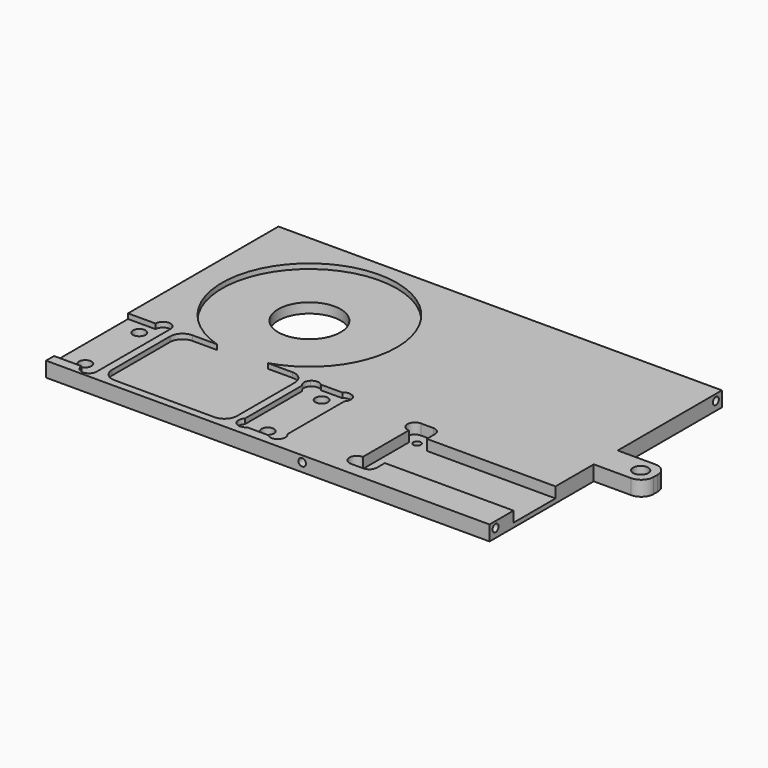
from build123d import *

# Parameters (mm, degrees)
F0_W      = 20
F0_H      = 12
F0_R      = 3
F1_DEPTH  = 6
F0_R_2    = 12.5
F0_R_3    = 2.5
F2_DEPTH  = 4
F3_DEPTH  = 2
F4_DEPTH  = 3
F0_R_4    = 1.5
F5_DEPTH  = 1.75
F6_R      = 1.5
F7_DEPTH  = 8
F8_R      = 1.5
F9_DEPTH  = 8
F10_R     = 1.5
F11_DEPTH = 5
F12_R     = 1.5
F13_DEPTH = 5
F14_R     = 5


# Not quite as in the source:
# - a feature names something its author has since deleted; it is built from what else it names


with BuildPart() as f1:
    # F0 (on Top) → F1 (new body)
    with BuildSketch(Plane.XY):
        with BuildLine():
            Line((0, 4), (0, 0))
            Line((0, 0), (177.5, 0))
            Line((177.5, 0), (177.5, 5))
            Line((177.5, 5), (177.5, 12))
            Line((177.5, 12), (126, 12))
            Line((126, 12), (126, 8))
            ThreePointArc((126, 8), (125.1213203436, 5.8786796564), (123, 5))
            Line((123, 5), (118, 5))
            ThreePointArc((118, 5), (115, 8), (118, 11))
            Line((118, 11), (118, 34))
            ThreePointArc((118, 34), (115, 37), (118, 40))
            Line((118, 40), (123, 40))
            ThreePointArc((123, 40), (125.1213203436, 39.1213203436), (126, 37))
            Line((126, 37), (126, 33))
            Line((126, 33), (177.5, 33))
            Line((177.5, 33), (177.5, 40))
            Line((177.5, 40), (177.5, 52.125))
            Line((177.5, 52.125), (177.5, 64.125))
            Line((177.5, 64.125), (177.5, 116.25))
            Line((177.5, 116.25), (0, 116.25))
            Line((0, 116.25), (0, 41))
            Line((0, 41), (11, 41))
            ThreePointArc((11, 41), (14, 44), (17, 41))
            Line((17, 41), (17, 4))
            ThreePointArc((17, 4), (14, 1), (11, 4))
            Line((11, 4), (0, 4))
        make_face()
        with BuildLine():
            Line((73, 8.2426406871), (73, 36.7573593129))
            ThreePointArc((73, 36.7573593129), (72.1213203436, 38.8786796564), (73, 41))
            ThreePointArc((73, 41), (75.1213203436, 41.8786796564), (77.2426406871, 41))
            Line((77.2426406871, 41), (85.7573593129, 41))
            ThreePointArc((85.7573593129, 41), (87.8786796564, 41.8786796564), (90, 41))
            ThreePointArc((90, 41), (90.8786796564, 38.8786796564), (90, 36.7573593129))
            Line((90, 36.7573593129), (90, 8.2426406871))
            ThreePointArc((90, 8.2426406871), (90.8786796564, 6.1213203436), (90, 4))
            ThreePointArc((90, 4), (87.8786796564, 3.1213203436), (85.7573593129, 4))
            Line((85.7573593129, 4), (77.2426406871, 4))
            ThreePointArc((77.2426406871, 4), (75.1213203436, 3.1213203436), (73, 4))
            ThreePointArc((73, 4), (72.1213203436, 6.1213203436), (73, 8.2426406871))
        make_face(mode=Mode.SUBTRACT)
        with BuildLine():
            ThreePointArc((34.8634325336, 42), (24.1407078419, 103.6049805312), (80, 75.5))
            ThreePointArc((80, 75.5), (73.1049805312, 54.6407078419), (55.1365674664, 42))
            Line((55.1365674664, 42), (65, 42))
            ThreePointArc((65, 42), (68.5355339059, 40.5355339059), (70, 37))
            Line((70, 37), (70, 8))
            ThreePointArc((70, 8), (68.5355339059, 4.4644660941), (65, 3))
            Line((65, 3), (25, 3))
            ThreePointArc((25, 3), (21.4644660941, 4.4644660941), (20, 8))
            Line((20, 8), (20, 37))
            ThreePointArc((20, 37), (21.4644660941, 40.5355339059), (25, 42))
            Line((25, 42), (34.8634325336, 42))
        make_face(mode=Mode.SUBTRACT)
        with Locations((187.5, 58.125)):
            Rectangle(F0_W, F0_H)
        with Locations((191.5, 58.125)):
            Circle(F0_R, mode=Mode.SUBTRACT)
    extrude(amount=F1_DEPTH)

    # F0 (on Top) → F2 (join)
    with BuildSketch(Plane.XY):
        with BuildLine():
            Line((55.1365674664, 42), (34.8634325336, 42))
            ThreePointArc((34.8634325336, 42), (45, 40.5), (55.1365674664, 42))
        make_face()
        with BuildLine():
            ThreePointArc((55.1365674664, 42), (73.1049805312, 54.6407078419), (80, 75.5))
            ThreePointArc((80, 75.5), (24.1407078419, 103.6049805312), (34.8634325336, 42))
            Line((34.8634325336, 42), (55.1365674664, 42))
        make_face()
        with Locations((45, 75.5)):
            Circle(F0_R_2, mode=Mode.SUBTRACT)
        with BuildLine():
            Line((0, 41), (0, 4))
            Line((0, 4), (11, 4))
            ThreePointArc((11, 4), (14, 1), (17, 4))
            Line((17, 4), (17, 41))
            ThreePointArc((17, 41), (14, 44), (11, 41))
            Line((11, 41), (0, 41))
        make_face()
        with Locations((8.5, 9)):
            Circle(F0_R_3, mode=Mode.SUBTRACT)
        with Locations((8.5, 36)):
            Circle(F0_R_3, mode=Mode.SUBTRACT)
        with BuildLine():
            ThreePointArc((73, 41), (72.1213203436, 38.8786796564), (73, 36.7573593129))
            Line((73, 36.7573593129), (73, 8.2426406871))
            ThreePointArc((73, 8.2426406871), (72.1213203436, 6.1213203436), (73, 4))
            ThreePointArc((73, 4), (75.1213203436, 3.1213203436), (77.2426406871, 4))
            Line((77.2426406871, 4), (85.7573593129, 4))
            ThreePointArc((85.7573593129, 4), (87.8786796564, 3.1213203436), (90, 4))
            ThreePointArc((90, 4), (90.8786796564, 6.1213203436), (90, 8.2426406871))
            Line((90, 8.2426406871), (90, 36.7573593129))
            ThreePointArc((90, 36.7573593129), (90.8786796564, 38.8786796564), (90, 41))
            ThreePointArc((90, 41), (87.8786796564, 41.8786796564), (85.7573593129, 41))
            Line((85.7573593129, 41), (77.2426406871, 41))
            ThreePointArc((77.2426406871, 41), (75.1213203436, 41.8786796564), (73, 41))
        make_face()
        with Locations((81.5, 9)):
            Circle(F0_R_3, mode=Mode.SUBTRACT)
        with Locations((81.5, 36)):
            Circle(F0_R_3, mode=Mode.SUBTRACT)
        with BuildLine():
            ThreePointArc((55.1365674664, 42), (45, 40.5), (34.8634325336, 42))
            Line((34.8634325336, 42), (25, 42))
            ThreePointArc((25, 42), (21.4644660941, 40.5355339059), (20, 37))
            Line((20, 37), (20, 8))
            ThreePointArc((20, 8), (21.4644660941, 4.4644660941), (25, 3))
            Line((25, 3), (65, 3))
            ThreePointArc((65, 3), (68.5355339059, 4.4644660941), (70, 8))
            Line((70, 8), (70, 37))
            ThreePointArc((70, 37), (68.5355339059, 40.5355339059), (65, 42))
            Line((65, 42), (55.1365674664, 42))
        make_face()
    extrude(amount=F2_DEPTH)

    # F0 (on Top) → F3 (join)
    with BuildSketch(Plane.XY):
        with BuildLine():
            ThreePointArc((55.1365674664, 42), (45, 40.5), (34.8634325336, 42))
            Line((34.8634325336, 42), (25, 42))
            ThreePointArc((25, 42), (21.4644660941, 40.5355339059), (20, 37))
            Line((20, 37), (20, 8))
            ThreePointArc((20, 8), (21.4644660941, 4.4644660941), (25, 3))
            Line((25, 3), (65, 3))
            ThreePointArc((65, 3), (68.5355339059, 4.4644660941), (70, 8))
            Line((70, 8), (70, 37))
            ThreePointArc((70, 37), (68.5355339059, 40.5355339059), (65, 42))
            Line((65, 42), (55.1365674664, 42))
        make_face()
    extrude(amount=F3_DEPTH)

    # F0 (on Top) → F4 (join)
    with BuildSketch(Plane.XY):
        with BuildLine():
            Line((0, 41), (0, 4))
            Line((0, 4), (11, 4))
            ThreePointArc((11, 4), (14, 1), (17, 4))
            Line((17, 4), (17, 41))
            ThreePointArc((17, 41), (14, 44), (11, 41))
            Line((11, 41), (0, 41))
        make_face()
        with Locations((8.5, 9)):
            Circle(F0_R_3, mode=Mode.SUBTRACT)
        with Locations((8.5, 36)):
            Circle(F0_R_3, mode=Mode.SUBTRACT)
        with BuildLine():
            Line((0, 4), (0, 0))
            Line((0, 0), (177.5, 0))
            Line((177.5, 0), (177.5, 5))
            Line((177.5, 5), (177.5, 12))
            Line((177.5, 12), (126, 12))
            Line((126, 12), (126, 8))
            ThreePointArc((126, 8), (125.1213203436, 5.8786796564), (123, 5))
            Line((123, 5), (118, 5))
            ThreePointArc((118, 5), (115, 8), (118, 11))
            Line((118, 11), (118, 34))
            ThreePointArc((118, 34), (115, 37), (118, 40))
            Line((118, 40), (123, 40))
            ThreePointArc((123, 40), (125.1213203436, 39.1213203436), (126, 37))
            Line((126, 37), (126, 33))
            Line((126, 33), (177.5, 33))
            Line((177.5, 33), (177.5, 40))
            Line((177.5, 40), (177.5, 52.125))
            Line((177.5, 52.125), (177.5, 64.125))
            Line((177.5, 64.125), (177.5, 116.25))
            Line((177.5, 116.25), (0, 116.25))
            Line((0, 116.25), (0, 41))
            Line((0, 41), (11, 41))
            ThreePointArc((11, 41), (14, 44), (17, 41))
            Line((17, 41), (17, 4))
            ThreePointArc((17, 4), (14, 1), (11, 4))
            Line((11, 4), (0, 4))
        make_face()
        with BuildLine():
            Line((73, 8.2426406871), (73, 36.7573593129))
            ThreePointArc((73, 36.7573593129), (72.1213203436, 38.8786796564), (73, 41))
            ThreePointArc((73, 41), (75.1213203436, 41.8786796564), (77.2426406871, 41))
            Line((77.2426406871, 41), (85.7573593129, 41))
            ThreePointArc((85.7573593129, 41), (87.8786796564, 41.8786796564), (90, 41))
            ThreePointArc((90, 41), (90.8786796564, 38.8786796564), (90, 36.7573593129))
            Line((90, 36.7573593129), (90, 8.2426406871))
            ThreePointArc((90, 8.2426406871), (90.8786796564, 6.1213203436), (90, 4))
            ThreePointArc((90, 4), (87.8786796564, 3.1213203436), (85.7573593129, 4))
            Line((85.7573593129, 4), (77.2426406871, 4))
            ThreePointArc((77.2426406871, 4), (75.1213203436, 3.1213203436), (73, 4))
            ThreePointArc((73, 4), (72.1213203436, 6.1213203436), (73, 8.2426406871))
        make_face(mode=Mode.SUBTRACT)
        with BuildLine():
            ThreePointArc((34.8634325336, 42), (24.1407078419, 103.6049805312), (80, 75.5))
            ThreePointArc((80, 75.5), (73.1049805312, 54.6407078419), (55.1365674664, 42))
            Line((55.1365674664, 42), (65, 42))
            ThreePointArc((65, 42), (68.5355339059, 40.5355339059), (70, 37))
            Line((70, 37), (70, 8))
            ThreePointArc((70, 8), (68.5355339059, 4.4644660941), (65, 3))
            Line((65, 3), (25, 3))
            ThreePointArc((25, 3), (21.4644660941, 4.4644660941), (20, 8))
            Line((20, 8), (20, 37))
            ThreePointArc((20, 37), (21.4644660941, 40.5355339059), (25, 42))
            Line((25, 42), (34.8634325336, 42))
        make_face(mode=Mode.SUBTRACT)
    extrude(amount=F4_DEPTH)

    # F0 (on Top) → F5 (join)
    with BuildSketch(Plane.XY):
        with BuildLine():
            Line((126, 12), (177.5, 12))
            Line((177.5, 12), (177.5, 33))
            Line((177.5, 33), (126, 33))
            Line((126, 33), (126, 37))
            ThreePointArc((126, 37), (125.1213203436, 39.1213203436), (123, 40))
            Line((123, 40), (118, 40))
            ThreePointArc((118, 40), (115, 37), (118, 34))
            Line((118, 34), (118, 11))
            ThreePointArc((118, 11), (115, 8), (118, 5))
            Line((118, 5), (123, 5))
            ThreePointArc((123, 5), (125.1213203436, 5.8786796564), (126, 8))
            Line((126, 8), (126, 12))
        make_face()
        with Locations((120.5, 10)):
            Circle(F0_R_4, mode=Mode.SUBTRACT)
        with Locations((120.5, 35)):
            Circle(F0_R_4, mode=Mode.SUBTRACT)
    extrude(amount=F5_DEPTH)

    # F6 (on face) → F7 (cut)
    with BuildSketch(Plane.YZ.offset(177.5)):
        with Locations((3, 3.5)):
            Circle(F6_R)
        with Locations((113.25, 3.5)):
            Circle(F6_R)
    extrude(amount=-F7_DEPTH, mode=Mode.SUBTRACT)

    # F8 (on face) → F9 (cut)
    with BuildSketch(Plane(origin=(0, 0, 0), x_dir=(0, -1, 0), z_dir=(-1, 0, 0))):
        with Locations((-113.25, 3.5)):
            Circle(F8_R)
        with Locations((-58.125, 3.5)):
            Circle(F8_R)
    extrude(amount=-F9_DEPTH, mode=Mode.SUBTRACT)

    # F10 (on face) → F11 (cut)
    with BuildSketch(Plane.XZ):
        with Locations((102.5, 3.5)):
            Circle(F10_R)
    extrude(amount=-F11_DEPTH, mode=Mode.SUBTRACT)

    # F12 (on face) → F13 (cut)
    with BuildSketch(Plane(origin=(0, 116.25, 0), x_dir=(-1, 0, 0), z_dir=(0, 1, 0))):
        with Locations((-88.75, 3.5)):
            Circle(F12_R)
    extrude(amount=-F13_DEPTH, mode=Mode.SUBTRACT)

    # F14
    f14_edges = [f1.edges().sort_by_distance(p)[0] for p in [
        (197.5, 52.125, 3),
        (197.5, 64.125, 3),
    ]]
    fillet(f14_edges, radius=F14_R)


solid = f1.part
